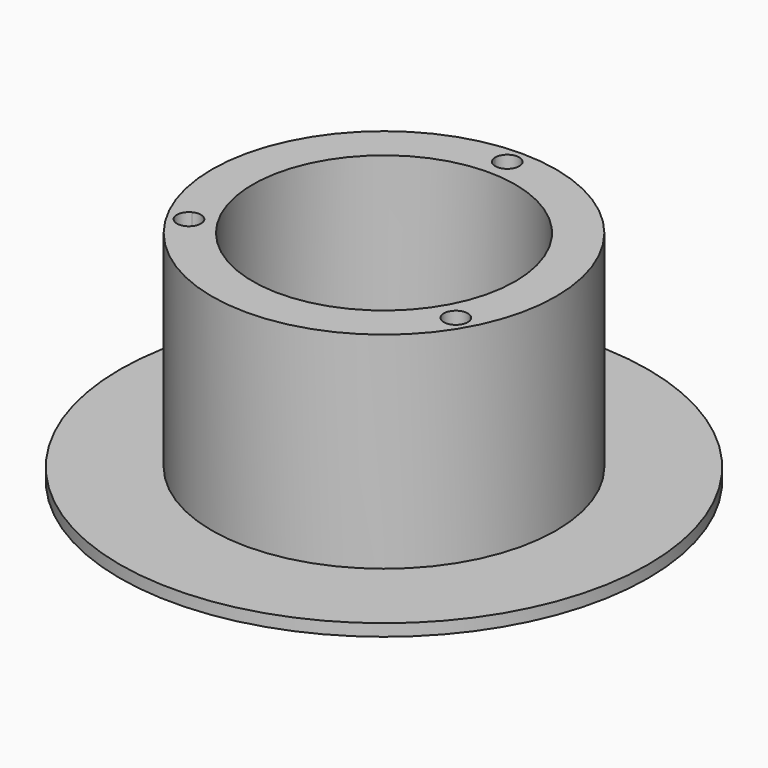
from build123d import *

# Parameters (mm, degrees)
F0_R     = 33
F0_R_2   = 21.5
F1_DEPTH = 1.5
F0_R_3   = 16.4
F2_DEPTH = 27.25
F0_R_4   = 14.2
F3_DEPTH = 2
F4_DEPTH = 21.5
F5_SIZE2 = 1.5
F5_SIZE  = 2


with BuildPart() as f1:
    # F0 (on Top) → F1 (new body)
    with BuildSketch(Plane.XY):
        Circle(F0_R)
        Circle(F0_R_2, mode=Mode.SUBTRACT)
    extrude(amount=F1_DEPTH)

    # F0 (on Top) → F2 (join)
    with BuildSketch(Plane.XY):
        Circle(F0_R_2)
        with BuildLine():
            ThreePointArc((1.4988610957, 19.1915584416), (14.1318005946, 13.0711404228), (19.25, 0))
            ThreePointArc((19.25, 0), (18.7740685276, -4.2540393653), (17.3698076965, -8.2977274351))
            ThreePointArc((17.3698076965, -8.2977274351), (17.9551673614, -8.8498316346), (18.1709890229, -9.625))
            ThreePointArc((18.1709890229, -9.625), (17.3955359043, -10.938404666), (15.8709466007, -10.8938310064))
            ThreePointArc((15.8709466007, -10.8938310064), (0, -19.25), (-15.8709466007, -10.8938310064))
            ThreePointArc((-15.8709466007, -10.8938310064), (-17.9700271285, -10.375), (-17.3698076965, -8.2977274351))
            ThreePointArc((-17.3698076965, -8.2977274351), (-16.6709890229, 9.625), (-1.4988610957, 19.1915584416))
            ThreePointArc((-1.4988610957, 19.1915584416), (-0.0292263274, 20.7497152469), (1.5, 19.25))
            ThreePointArc((1.5, 19.25), (1.4997152469, 19.2207736726), (1.4988610957, 19.1915584416))
        make_face(mode=Mode.SUBTRACT)
        with BuildLine():
            ThreePointArc((17.3698076965, -8.2977274351), (18.7740685276, -4.2540393653), (19.25, 0))
            ThreePointArc((19.25, 0), (14.1318005946, 13.0711404228), (1.4988610957, 19.1915584416))
            ThreePointArc((1.4988610957, 19.1915584416), (0, 17.75), (-1.4988610957, 19.1915584416))
            ThreePointArc((-1.4988610957, 19.1915584416), (-16.6709890229, 9.625), (-17.3698076965, -8.2977274351))
            ThreePointArc((-17.3698076965, -8.2977274351), (-15.8958206574, -8.3408216614), (-15.1709890229, -9.625))
            ThreePointArc((-15.1709890229, -9.625), (-15.3575843569, -10.3495468815), (-15.8709466007, -10.8938310064))
            ThreePointArc((-15.8709466007, -10.8938310064), (0, -19.25), (15.8709466007, -10.8938310064))
            ThreePointArc((15.8709466007, -10.8938310064), (15.3719509172, -8.875), (17.3698076965, -8.2977274351))
        make_face()
        Circle(F0_R_3, mode=Mode.SUBTRACT)
    extrude(amount=F2_DEPTH)

    # F0 (on Top) → F3 (join)
    with BuildSketch(Plane.XY):
        Circle(F0_R_3)
        Circle(F0_R_4, mode=Mode.SUBTRACT)
    extrude(amount=F3_DEPTH)

    # F0 (on Top) → F4 (join)
    with BuildSketch(Plane.XY):
        Circle(F0_R_2)
        with BuildLine():
            ThreePointArc((1.4988610957, 19.1915584416), (14.1318005946, 13.0711404228), (19.25, 0))
            ThreePointArc((19.25, 0), (18.7740685276, -4.2540393653), (17.3698076965, -8.2977274351))
            ThreePointArc((17.3698076965, -8.2977274351), (17.9551673614, -8.8498316346), (18.1709890229, -9.625))
            ThreePointArc((18.1709890229, -9.625), (17.3955359043, -10.938404666), (15.8709466007, -10.8938310064))
            ThreePointArc((15.8709466007, -10.8938310064), (0, -19.25), (-15.8709466007, -10.8938310064))
            ThreePointArc((-15.8709466007, -10.8938310064), (-17.9700271285, -10.375), (-17.3698076965, -8.2977274351))
            ThreePointArc((-17.3698076965, -8.2977274351), (-16.6709890229, 9.625), (-1.4988610957, 19.1915584416))
            ThreePointArc((-1.4988610957, 19.1915584416), (-0.0292263274, 20.7497152469), (1.5, 19.25))
            ThreePointArc((1.5, 19.25), (1.4997152469, 19.2207736726), (1.4988610957, 19.1915584416))
        make_face(mode=Mode.SUBTRACT)
        with BuildLine():
            ThreePointArc((17.3698076965, -8.2977274351), (18.7740685276, -4.2540393653), (19.25, 0))
            ThreePointArc((19.25, 0), (14.1318005946, 13.0711404228), (1.4988610957, 19.1915584416))
            ThreePointArc((1.4988610957, 19.1915584416), (0, 17.75), (-1.4988610957, 19.1915584416))
            ThreePointArc((-1.4988610957, 19.1915584416), (-16.6709890229, 9.625), (-17.3698076965, -8.2977274351))
            ThreePointArc((-17.3698076965, -8.2977274351), (-15.8958206574, -8.3408216614), (-15.1709890229, -9.625))
            ThreePointArc((-15.1709890229, -9.625), (-15.3575843569, -10.3495468815), (-15.8709466007, -10.8938310064))
            ThreePointArc((-15.8709466007, -10.8938310064), (0, -19.25), (15.8709466007, -10.8938310064))
            ThreePointArc((15.8709466007, -10.8938310064), (15.3719509172, -8.875), (17.3698076965, -8.2977274351))
        make_face()
        Circle(F0_R_3, mode=Mode.SUBTRACT)
        with BuildLine():
            ThreePointArc((-1.4988610957, 19.1915584416), (0, 19.25), (1.4988610957, 19.1915584416))
            ThreePointArc((1.4988610957, 19.1915584416), (1.4997152469, 19.2207736726), (1.5, 19.25))
            ThreePointArc((1.5, 19.25), (-0.0292263274, 20.7497152469), (-1.4988610957, 19.1915584416))
        make_face()
        with BuildLine():
            ThreePointArc((18.1709890229, -9.625), (17.9551673614, -8.8498316346), (17.3698076965, -8.2977274351))
            ThreePointArc((17.3698076965, -8.2977274351), (16.6709890229, -9.625), (15.8709466007, -10.8938310064))
            ThreePointArc((15.8709466007, -10.8938310064), (17.3955359043, -10.938404666), (18.1709890229, -9.625))
        make_face()
        with BuildLine():
            ThreePointArc((-15.8709466007, -10.8938310064), (-16.6709890229, -9.625), (-17.3698076965, -8.2977274351))
            ThreePointArc((-17.3698076965, -8.2977274351), (-17.9700271285, -10.375), (-15.8709466007, -10.8938310064))
        make_face()
        with BuildLine():
            ThreePointArc((-1.4988610957, 19.1915584416), (0, 17.75), (1.4988610957, 19.1915584416))
            ThreePointArc((1.4988610957, 19.1915584416), (0, 19.25), (-1.4988610957, 19.1915584416))
        make_face()
        with BuildLine():
            ThreePointArc((15.8709466007, -10.8938310064), (16.6709890229, -9.625), (17.3698076965, -8.2977274351))
            ThreePointArc((17.3698076965, -8.2977274351), (15.3719509172, -8.875), (15.8709466007, -10.8938310064))
        make_face()
        with BuildLine():
            ThreePointArc((-15.1709890229, -9.625), (-15.8958206574, -8.3408216614), (-17.3698076965, -8.2977274351))
            ThreePointArc((-17.3698076965, -8.2977274351), (-16.6709890229, -9.625), (-15.8709466007, -10.8938310064))
            ThreePointArc((-15.8709466007, -10.8938310064), (-15.3575843569, -10.3495468815), (-15.1709890229, -9.625))
        make_face()
    extrude(amount=F4_DEPTH)

    # F5
    f5_edges = [f1.edges().sort_by_distance(p)[0] for p in [
        (-14.2, 0, 0),
    ]]
    f5_side = f1.faces().sort_by_distance((-32.066619, 0, 0))[0]
    chamfer(f5_edges, length=F5_SIZE, length2=F5_SIZE2, reference=f5_side)


solid = f1.part
